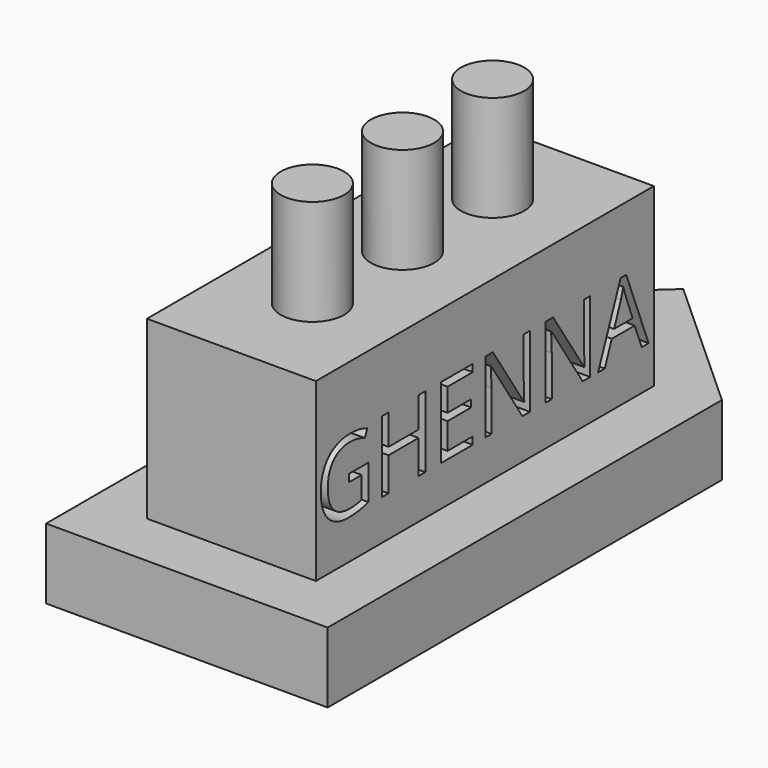
from build123d import *

# Parameters (mm, degrees)
F1_DEPTH     = 10
F2_W         = 24
F2_H         = 60
F3_DEPTH     = 25
F4_R         = 4.5
F5_DEPTH     = 15
F7_TEXT_SIZE = 14.1933099242
F8_DEPTH     = 5
F6_TEXT_SIZE = 11.6178806444
F9_DEPTH     = 5


# Not quite as in the source:
# - Text() gives the source's letters only with a copy of the font that has no kerning and outlines rounded to 1/6400 em; it was checked with that copy


with BuildPart() as f1:
    # F0 (on Top) → F1 (new body)
    with BuildSketch(Plane.XY):
        Polygon((0, 39.2941792635), (-20, 21.1558221163), (-20, -48.8441778837), (20, -48.8441778837), (20, 21.1558221163), align=None)
    extrude(amount=F1_DEPTH)

    # F2 (on face) → F3 (join)
    with BuildSketch(Plane.XY.offset(10)):
        with Locations((0, -10.9349852658)):
            Rectangle(F2_W, F2_H)
    extrude(amount=F3_DEPTH)

    # F7 (on face) → F8 (cut)
    with BuildSketch(Plane.YZ.offset(12)):
        with Locations((-40.9349852658, 15.714600102)):
            Text('GHENNA', F7_TEXT_SIZE, font='Open Sans', text_align=(TextAlign.LEFT, TextAlign.BOTTOM))
    extrude(amount=-F8_DEPTH, mode=Mode.SUBTRACT)

    # F6 (on face) → F9 (cut)
    with BuildSketch(Plane(origin=(-12, 0, 0), x_dir=(0, -1, 0), z_dir=(-1, 0, 0))):
        with Locations((-8.1139282216, 17.7318919593)):
            Text('NUJOD', F6_TEXT_SIZE, font='Open Sans', font_style=FontStyle.BOLD, text_align=(TextAlign.LEFT, TextAlign.BOTTOM))
    extrude(amount=-F9_DEPTH, mode=Mode.SUBTRACT)


with BuildPart() as f5:
    # F4 (on face) → F5 (new body)
    with BuildSketch(Plane.XY.offset(35)):
        with Locations((0, 5.440727219)):
            Circle(F4_R)
    extrude(amount=F5_DEPTH)


with BuildPart() as f5b:
    # F4 (on face) → F5, piece 2 (new body)
    with BuildSketch(Plane.XY.offset(35)):
        with Locations((0, -10.559272781)):
            Circle(F4_R)
    extrude(amount=F5_DEPTH)


with BuildPart() as f5c:
    # F4 (on face) → F5, piece 3 (new body)
    with BuildSketch(Plane.XY.offset(35)):
        with Locations((0, -26.559272781)):
            Circle(F4_R)
    extrude(amount=F5_DEPTH)


solid = Compound([f1.part, f5.part, f5b.part, f5c.part])
